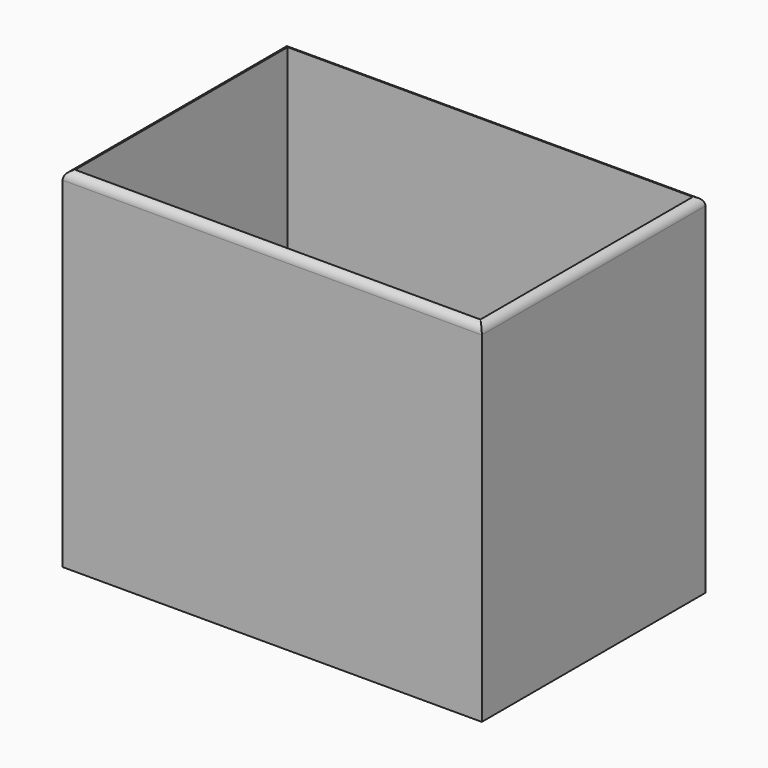
from build123d import *

# Parameters (mm, degrees)
F0_W        = 152.4
F0_H        = 101.6
F1_DEPTH    = 127
F2_T        = -2.54
F3_T1_DEPTH = 117.475
F3_T3_DEPTH = 168.275


# Not quite as in the source:
# - a fillet or chamfer that OpenCascade refuses, or shapes differently, is made with other operations: its cross-section is extruded or revolved along the edge and cut away or added


with BuildPart() as f1:
    # F0 (on Top) → F1 (new body)
    with BuildSketch(Plane.XY):
        with Locations((76.2, 50.8)):
            Rectangle(F0_W, F0_H)
    extrude(amount=F1_DEPTH)

    # F2
    f2_openings = [f1.faces().sort_by_distance(p)[0] for p in [
        (76.2, 50.8, 127),
    ]]
    offset(amount=F2_T, openings=f2_openings)

    # F3: fillet of radius 3.175 on 4 edges, made by hand

    # F3_s2 → F3_t1 (cut)
    with BuildSketch(Plane.XZ.offset(-109.5375)):
        with BuildLine():
            ThreePointArc((0, 123.825), (0.9299359697, 126.0700640303), (3.175, 127))
            Line((3.175, 127), (0, 127))
            Line((0, 127), (0, 123.825))
        make_face()
        with BuildLine():
            ThreePointArc((152.4, 123.825), (151.4700640303, 126.0700640303), (149.225, 127))
            Line((149.225, 127), (152.4, 127))
            Line((152.4, 127), (152.4, 123.825))
        make_face()
    extrude(amount=F3_T1_DEPTH, mode=Mode.SUBTRACT)

    # F3_s4 → F3_t3 (cut)
    with BuildSketch(Plane.YZ.offset(-7.9375)):
        with BuildLine():
            ThreePointArc((0, 123.825), (0.9299359697, 126.0700640303), (3.175, 127))
            Line((3.175, 127), (0, 127))
            Line((0, 127), (0, 123.825))
        make_face()
        with BuildLine():
            ThreePointArc((101.6, 123.825), (100.6700640303, 126.0700640303), (98.425, 127))
            Line((98.425, 127), (101.6, 127))
            Line((101.6, 127), (101.6, 123.825))
        make_face()
    extrude(amount=F3_T3_DEPTH, mode=Mode.SUBTRACT)


solid = f1.part
